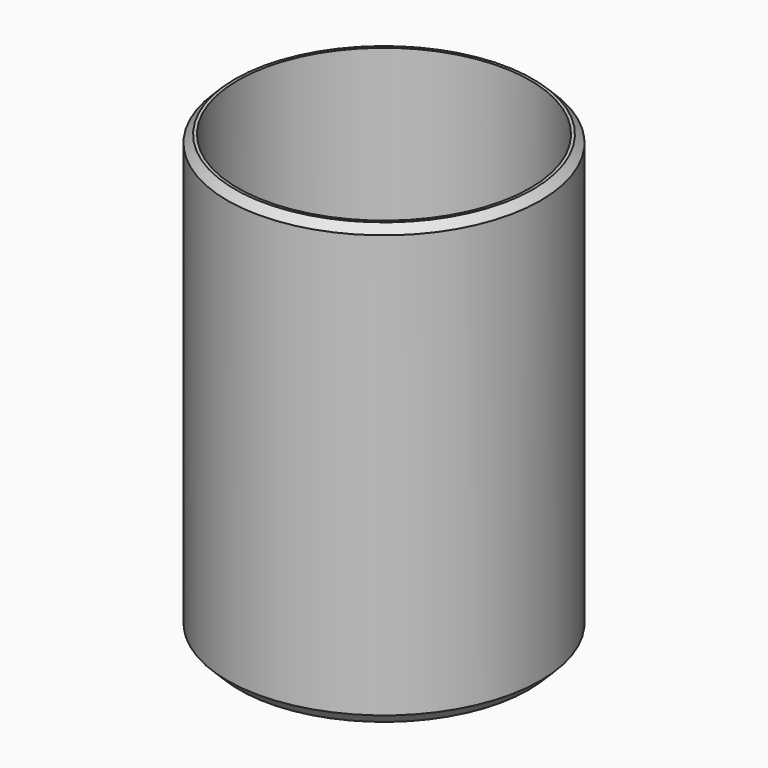
from build123d import *

# Parameters (mm, degrees)
F0_R     = 9.75
F1_DEPTH = 0.5
F0_R_2   = 10.45
F2_DEPTH = 29.5
F3_SIZE  = 0.5
F4_SIZE  = 0.4
F5_SIZE  = 0.8


with BuildPart() as f1:
    # F0 (on Top) → F1 (new body)
    with BuildSketch(Plane.XY):
        Circle(F0_R)
    extrude(amount=F1_DEPTH)

    # F0 (on Top) → F2 (join)
    with BuildSketch(Plane.XY):
        Circle(F0_R_2)
        Circle(F0_R, mode=Mode.SUBTRACT)
    extrude(amount=F2_DEPTH)

    # F3
    f3_edges = [f1.edges().sort_by_distance(p)[0] for p in [
        (-10.45, 0, 29.5),
    ]]
    chamfer(f3_edges, length=F3_SIZE)

    # F4
    f4_edges = [f1.edges().sort_by_distance(p)[0] for p in [
        (-9.75, 0, 0.5),
    ]]
    chamfer(f4_edges, length=F4_SIZE)

    # F5
    f5_edges = [f1.edges().sort_by_distance(p)[0] for p in [
        (-10.45, 0, 0),
    ]]
    chamfer(f5_edges, length=F5_SIZE)


solid = f1.part
